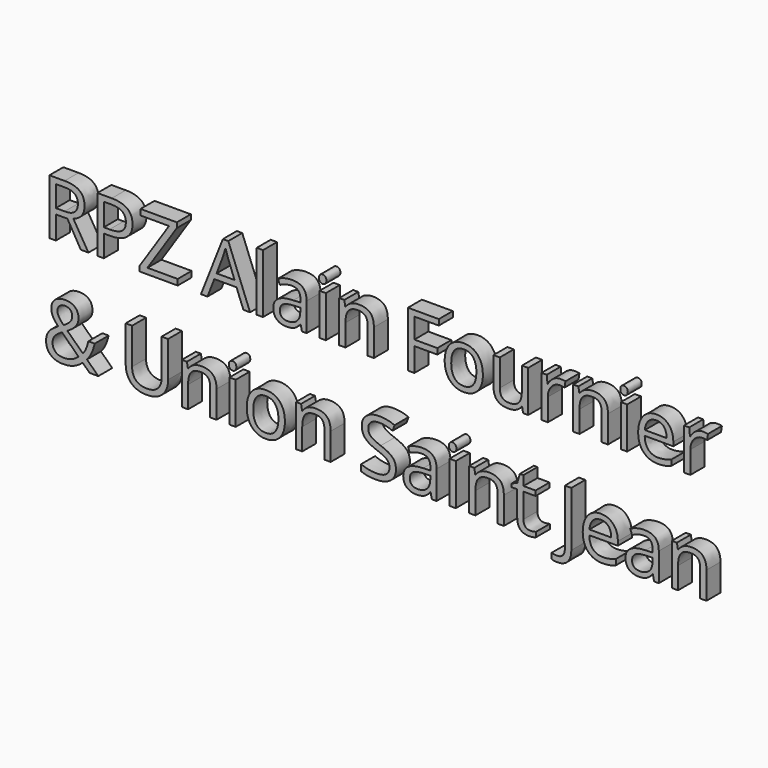
from build123d import *

# Parameters (mm, degrees)
F0_TEXT_SIZE = 33.8735835006
F1_DEPTH     = 7.62


# Not quite as in the source:
# - Text() gives the source's letters only with a copy of the font that has no kerning and outlines rounded to 1/6400 em; it was checked with that copy


with BuildPart() as f1:
    # F0 (on Front) → F1 (new body)
    with BuildSketch(Plane.XZ):
        with Locations((-125.4237443209, 34.6740782261)):
            Text('RPZ Alain Fournier', F0_TEXT_SIZE, font='Open Sans', text_align=(TextAlign.LEFT, TextAlign.BOTTOM))
        with Locations((-125.4237443209, -11.3939953347)):
            Text('& Union Saint Jean', F0_TEXT_SIZE, font='Open Sans', text_align=(TextAlign.LEFT, TextAlign.BOTTOM))
    extrude(amount=F1_DEPTH)


solid = f1.part
